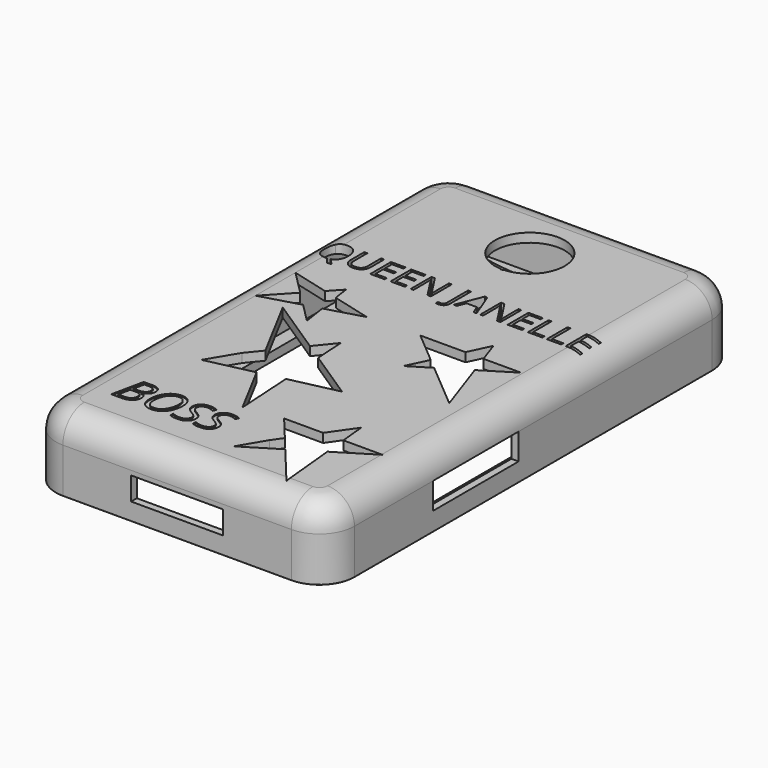
from build123d import *

# Parameters (mm, degrees)
F0_W          = 63.5
F0_H          = 112.33
F1_DEPTH      = 2
F2_W          = 63.5
F2_H          = 112.33
F3_DEPTH      = 14
F3_DEPTH_BACK = 2
F4_T1_DEPTH   = 96.7
F4_T3_DEPTH   = 145.53
F5_R          = 6.935383727
F6_T1_DEPTH   = 35.5580872669
F6_T4_ANGLE   = 90
F6_T6_ANGLE   = 90
F6_T8_ANGLE   = 90
F6_T10_ANGLE  = 90
F7_W          = 20.5546487123
F7_H          = 5.1386626437
F8_DEPTH      = 3
F9_W          = 23.8308350714
F9_H          = 5.891926311
F10_DEPTH     = 3
F11_R         = 0.0241421356
F12_W         = 98.4592325459
F12_H         = 2
F13_DEPTH     = 3
F14_SIZE2     = 2.99999
F14_SIZE      = 2.99999
F15_W         = 98.4592325459
F15_H         = 2
F16_DEPTH     = 3
F17_T1_DEPTH  = 41.9217985567
F18_W         = 49.6292325459
F18_H         = 2
F19_DEPTH     = 2
F20_T1_DEPTH  = 34.7871926215
F21_W         = 49.6292325459
F21_H         = 2
F22_DEPTH     = 2
F23_T1_DEPTH  = 68.0060422667
F24_TEXT_SIZE = 10.0512456562
F25_DEPTH     = 0.25


# Not quite as in the source:
# - a fillet or chamfer that OpenCascade refuses, or shapes differently, is made with other operations: its cross-section is extruded or revolved along the edge and cut away or added
# - a fillet or chamfer is up to 0.001 mm smaller than in the source, because OpenCascade refuses the exact size
# - Text() gives the source's letters only with a copy of the font that has no kerning and outlines rounded to 1/6400 em; it was checked with that copy


with BuildPart() as f1:
    # F0 (on Top) → F1 (new body)
    with BuildSketch(Plane.XY):
        Rectangle(F0_W, F0_H)
        Polygon((-19.5567887276, -26.5271142125), (-15.6769864261, -20.0607776642), (-13.0461571128, -16.8181271141), (-20.8500549197, -2.2136894986), (-8.0333166388, -10.6395088974), (-4.5548896305, -6.3521447591), (-4.1380456231, -13.200289134), (7.0845154114, -20.5780845135), (-3.5444898727, -22.95155196), (-2.7443135623, -36.097291857), (-9.1052395952, -24.1932729011), align=None, mode=Mode.SUBTRACT)
        Polygon((5.2739456296, -48.5126599669), (8.6364364251, -42.822279036), (10.2551206137, -40.5036243665), (5.5325948633, -34.8040238023), (14.2340888646, -34.8040238023), (18.2066168636, -29.1136484593), (18.7632836633, -34.8040238023), (27.5181401521, -34.8040238023), (19.2610861883, -39.8926750666), (20.5344967544, -52.9097691178), (12.9642616027, -43.7732775829), align=None, mode=Mode.SUBTRACT)
        Polygon((14.0059814319, -3.5149313177), (9.4123966992, -6.3521447591), (11.6904901042, -1.5602956646), (4.4979848899, 4.5113000087), (14.5769879443, 4.5113000087), (16.9133506715, 9.4257155433), (18.6099937738, 4.5113000087), (27.0008351654, 4.5113000087), (20.0847471782, 0.2395995958), (24.4142990559, -12.3011739925), align=None, mode=Mode.SUBTRACT)
        Polygon((-18.7007825335, 0.7888890234), (-27.316392865, -1.6963831149), (-21.9534791663, 4.049595339), (-27.3163933307, 9.4257155433), (-18.9805437499, 7.234883003), (-16.4529476315, 9.9430214614), (-15.9208933132, 6.4307440038), (-7.141424343, 4.1233191732), (-15.2184121265, 1.7934189192), (-14.4154893138, -3.506956622), align=None, mode=Mode.SUBTRACT)
        with BuildLine():
            add(Edge.make_bspline(
                [(-24.7315613885, 22.2938555124), (-24.029910942, 21.5008509389), (-24.029910942, 20.1051628897)],
                knots=[0, 0, 0, 1, 1, 1], degree=2))
            add(Edge.make_bspline(
                [(-24.029910942, 20.1051628897), (-24.029910942, 18.991150065), (-24.477799925, 18.2533386099)],
                knots=[0, 0, 0, 1, 1, 1], degree=2))
            add(Edge.make_bspline(
                [(-24.477799925, 18.2533386099), (-24.9256889081, 17.5155271547), (-25.7428008206, 17.2541528473)],
                knots=[0, 0, 0, 1, 1, 1], degree=2))
            Line((-25.7428008206, 17.2541528473), (-24.3636072665, 15.817862964))
            Line((-24.3636072665, 15.817862964), (-25.3431265156, 15.817862964))
            Line((-25.3431265156, 15.817862964), (-26.4723650281, 17.1272721156))
            Line((-26.4723650281, 17.1272721156), (-26.6905998867, 17.1183904644))
            add(Edge.make_bspline(
                [(-26.6905998867, 17.1183904644), (-27.9708264701, 17.1183904644), (-28.6667672837, 17.9018789829)],
                knots=[0, 0, 0, 1, 1, 1], degree=2))
            add(Edge.make_bspline(
                [(-28.6667672837, 17.9018789829), (-29.3627080973, 18.6853675015), (-29.3627080973, 20.1127757336)],
                knots=[0, 0, 0, 1, 1, 1], degree=2))
            add(Edge.make_bspline(
                [(-29.3627080973, 20.1127757336), (-29.3627080973, 21.5287646999), (-28.6648640727, 22.3078123929)],
                knots=[0, 0, 0, 1, 1, 1], degree=2))
            add(Edge.make_bspline(
                [(-28.6648640727, 22.3078123929), (-27.9670200481, 23.0868600858), (-26.6829870428, 23.0868600858)],
                knots=[0, 0, 0, 1, 1, 1], degree=2))
            add(Edge.make_bspline(
                [(-26.6829870428, 23.0868600858), (-25.4332118351, 23.0868600858), (-24.7315613885, 22.2938555124)],
                knots=[0, 0, 0, 1, 1, 1], degree=2))
        make_face(mode=Mode.SUBTRACT)
        with BuildLine():
            Line((-19.034616533, 22.9955059589), (-18.3608798475, 22.9955059589))
            Line((-18.3608798475, 22.9955059589), (-18.3608798475, 19.2449115285))
            add(Edge.make_bspline(
                [(-18.3608798475, 19.2449115285), (-18.3608798475, 18.2527042062), (-18.9597569013, 17.6855473353)],
                knots=[0, 0, 0, 1, 1, 1], degree=2))
            add(Edge.make_bspline(
                [(-18.9597569013, 17.6855473353), (-19.5586339552, 17.1183904644), (-20.6053999921, 17.1183904644)],
                knots=[0, 0, 0, 1, 1, 1], degree=2))
            add(Edge.make_bspline(
                [(-20.6053999921, 17.1183904644), (-21.652166029, 17.1183904644), (-22.2250325328, 17.6899881609)],
                knots=[0, 0, 0, 1, 1, 1], degree=2))
            add(Edge.make_bspline(
                [(-22.2250325328, 17.6899881609), (-22.7978990367, 18.2615858574), (-22.7978990367, 19.2601372163)],
                knots=[0, 0, 0, 1, 1, 1], degree=2))
            Line((-22.7978990367, 19.2601372163), (-22.7978990367, 22.9955059589))
            Line((-22.7978990367, 22.9955059589), (-22.1228935438, 22.9955059589))
            Line((-22.1228935438, 22.9955059589), (-22.1228935438, 19.2131913455))
            add(Edge.make_bspline(
                [(-22.1228935438, 19.2131913455), (-22.1228935438, 18.4874335599), (-21.7263912571, 18.0985441171)],
                knots=[0, 0, 0, 1, 1, 1], degree=2))
            add(Edge.make_bspline(
                [(-21.7263912571, 18.0985441171), (-21.3298889704, 17.7096546743), (-20.560991736, 17.7096546743)],
                knots=[0, 0, 0, 1, 1, 1], degree=2))
            add(Edge.make_bspline(
                [(-20.560991736, 17.7096546743), (-19.8276211065, 17.7096546743), (-19.4311188198, 18.1004473281)],
                knots=[0, 0, 0, 1, 1, 1], degree=2))
            add(Edge.make_bspline(
                [(-19.4311188198, 18.1004473281), (-19.034616533, 18.4912399819), (-19.034616533, 19.2208041894)],
                knots=[0, 0, 0, 1, 1, 1], degree=2))
            Line((-19.034616533, 19.2208041894), (-19.034616533, 22.9955059589))
        make_face(mode=Mode.SUBTRACT)
        Polygon((-13.595239563, 17.8010088012), (-13.595239563, 17.1983253254), (-16.8268918006, 17.1983253254), (-16.8268918006, 22.9955059589), (-13.595239563, 22.9955059589), (-13.595239563, 22.3966289051), (-16.1531551151, 22.3966289051), (-16.1531551151, 20.5289445338), (-13.7500340558, 20.5289445338), (-13.7500340558, 19.9338739019), (-16.1531551151, 19.9338739019), (-16.1531551151, 17.8010088012), align=None, mode=Mode.SUBTRACT)
        Polygon((-9.0795543201, 17.8010088012), (-9.0795543201, 17.1983253254), (-12.3112065577, 17.1983253254), (-12.3112065577, 22.9955059589), (-9.0795543201, 22.9955059589), (-9.0795543201, 22.3966289051), (-11.6374698722, 22.3966289051), (-11.6374698722, 20.5289445338), (-9.2343488128, 20.5289445338), (-9.2343488128, 19.9338739019), (-11.6374698722, 19.9338739019), (-11.6374698722, 17.8010088012), align=None, mode=Mode.SUBTRACT)
        with BuildLine():
            Line((-3.2671479987, 22.9955059589), (-3.2671479987, 17.1983253254))
            Line((-3.2671479987, 17.1983253254), (-4.0360452331, 17.1983253254))
            Line((-4.0360452331, 17.1983253254), (-7.2042571049, 22.0629325806))
            Line((-7.2042571049, 22.0629325806), (-7.2359772878, 22.0629325806))
            add(Edge.make_bspline(
                [(-7.2359772878, 22.0629325806), (-7.1725369219, 21.2064876413), (-7.1725369219, 20.4934179289)],
                knots=[0, 0, 0, 1, 1, 1], degree=2))
            Line((-7.1725369219, 20.4934179289), (-7.1725369219, 17.1983253254))
            Line((-7.1725369219, 17.1983253254), (-7.7955213148, 17.1983253254))
            Line((-7.7955213148, 17.1983253254), (-7.7955213148, 22.9955059589))
            Line((-7.7955213148, 22.9955059589), (-7.0342369243, 22.9955059589))
            Line((-7.0342369243, 22.9955059589), (-3.8736378965, 18.1499308135))
            Line((-3.8736378965, 18.1499308135), (-3.8419177136, 18.1499308135))
            add(Edge.make_bspline(
                [(-3.8419177136, 18.1499308135), (-3.8495305575, 18.2565106282), (-3.8774443185, 18.8376243796)],
                knots=[0, 0, 0, 1, 1, 1], degree=2))
            add(Edge.make_bspline(
                [(-3.8774443185, 18.8376243796), (-3.9053580794, 19.418738131), (-3.8977452355, 19.6686931725)],
                knots=[0, 0, 0, 1, 1, 1], degree=2))
            Line((-3.8977452355, 19.6686931725), (-3.8977452355, 22.9955059589))
            Line((-3.8977452355, 22.9955059589), (-3.2671479987, 22.9955059589))
        make_face(mode=Mode.SUBTRACT)
        with BuildLine():
            add(Edge.make_bspline(
                [(0.6864556025, 16.0862157116), (0.3058134073, 15.6719501224), (-0.4085251125, 15.6719501224)],
                knots=[0, 0, 0, 1, 1, 1], degree=2))
            add(Edge.make_bspline(
                [(-0.4085251125, 15.6719501224), (-0.7802856565, 15.6719501224), (-0.9947140931, 15.7785299371)],
                knots=[0, 0, 0, 1, 1, 1], degree=2))
            Line((-0.9947140931, 15.7785299371), (-0.9947140931, 16.3532996519))
            add(Edge.make_bspline(
                [(-0.9947140931, 16.3532996519), (-0.7130388687, 16.2746335983), (-0.4085251125, 16.2746335983)],
                knots=[0, 0, 0, 1, 1, 1], degree=2))
            add(Edge.make_bspline(
                [(-0.4085251125, 16.2746335983), (-0.015194844, 16.2746335983), (0.1890831341, 16.5125349703)],
                knots=[0, 0, 0, 1, 1, 1], degree=2))
            add(Edge.make_bspline(
                [(0.1890831341, 16.5125349703), (0.3933611122, 16.7504363423), (0.3933611122, 17.1983253254)],
                knots=[0, 0, 0, 1, 1, 1], degree=2))
            Line((0.3933611122, 17.1983253254), (0.3933611122, 22.9955059589))
            Line((0.3933611122, 22.9955059589), (1.0670977978, 22.9955059589))
            Line((1.0670977978, 22.9955059589), (1.0670977978, 17.2541528473))
            add(Edge.make_bspline(
                [(1.0670977978, 17.2541528473), (1.0670977978, 16.5004813008), (0.6864556025, 16.0862157116)],
                knots=[0, 0, 0, 1, 1, 1], degree=2))
        make_face(mode=Mode.SUBTRACT)
        Polygon((6.946750907, 17.1983253254), (6.2489068823, 17.1983253254), (5.5269555187, 19.0419023577), (3.2037693204, 19.0419023577), (2.490699608, 17.1983253254), (1.8080812712, 17.1983253254), (4.0995472865, 23.019613298), (4.6667041574, 23.019613298), align=None, mode=Mode.SUBTRACT)
        with BuildLine():
            Line((12.2719352184, 22.9955059589), (12.2719352184, 17.1983253254))
            Line((12.2719352184, 17.1983253254), (11.503037984, 17.1983253254))
            Line((11.503037984, 17.1983253254), (8.3348261123, 22.0629325806))
            Line((8.3348261123, 22.0629325806), (8.3031059293, 22.0629325806))
            add(Edge.make_bspline(
                [(8.3031059293, 22.0629325806), (8.3665462952, 21.2064876413), (8.3665462952, 20.4934179289)],
                knots=[0, 0, 0, 1, 1, 1], degree=2))
            Line((8.3665462952, 20.4934179289), (8.3665462952, 17.1983253254))
            Line((8.3665462952, 17.1983253254), (7.7435619023, 17.1983253254))
            Line((7.7435619023, 17.1983253254), (7.7435619023, 22.9955059589))
            Line((7.7435619023, 22.9955059589), (8.5048462928, 22.9955059589))
            Line((8.5048462928, 22.9955059589), (11.6654453207, 18.1499308135))
            Line((11.6654453207, 18.1499308135), (11.6971655036, 18.1499308135))
            add(Edge.make_bspline(
                [(11.6971655036, 18.1499308135), (11.6895526597, 18.2565106282), (11.6616388987, 18.8376243796)],
                knots=[0, 0, 0, 1, 1, 1], degree=2))
            add(Edge.make_bspline(
                [(11.6616388987, 18.8376243796), (11.6337251377, 19.418738131), (11.6413379816, 19.6686931725)],
                knots=[0, 0, 0, 1, 1, 1], degree=2))
            Line((11.6413379816, 19.6686931725), (11.6413379816, 22.9955059589))
            Line((11.6413379816, 22.9955059589), (12.2719352184, 22.9955059589))
        make_face(mode=Mode.SUBTRACT)
        Polygon((17.0972094468, 17.8010088012), (17.0972094468, 17.1983253254), (13.8655572092, 17.1983253254), (13.8655572092, 22.9955059589), (17.0972094468, 22.9955059589), (17.0972094468, 22.3966289051), (14.5392938947, 22.3966289051), (14.5392938947, 20.5289445338), (16.9424149541, 20.5289445338), (16.9424149541, 19.9338739019), (14.5392938947, 19.9338739019), (14.5392938947, 17.8010088012), align=None, mode=Mode.SUBTRACT)
        Polygon((21.6128946897, 17.1983253254), (18.3812424521, 17.1983253254), (18.3812424521, 22.9955059589), (19.0549791377, 22.9955059589), (19.0549791377, 17.8086216451), (21.6128946897, 17.8086216451), align=None, mode=Mode.SUBTRACT)
        Polygon((25.8278725984, 17.1983253254), (22.5962203607, 17.1983253254), (22.5962203607, 22.9955059589), (23.2699570463, 22.9955059589), (23.2699570463, 17.8086216451), (25.8278725984, 17.8086216451), align=None, mode=Mode.SUBTRACT)
        Polygon((30.042850507, 17.8010088012), (30.042850507, 17.1983253254), (26.8111982694, 17.1983253254), (26.8111982694, 22.9955059589), (30.042850507, 22.9955059589), (30.042850507, 22.3966289051), (27.484934955, 22.3966289051), (27.484934955, 20.5289445338), (29.8880560143, 20.5289445338), (29.8880560143, 19.9338739019), (27.484934955, 19.9338739019), (27.484934955, 17.8010088012), align=None, mode=Mode.SUBTRACT)
        with BuildLine():
            ThreePointArc((0.3612935402, 32.9422556185), (0, 32.765), (-0.3612935402, 32.9422556185))
            ThreePointArc((-0.3612935402, 32.9422556185), (-5.3783392405, 46.3566647828), (7.7889119618, 40.7227836549))
            ThreePointArc((7.7889119618, 40.7227836549), (5.6338811279, 35.3444444145), (0.3612935402, 32.9422556185))
        make_face(mode=Mode.SUBTRACT)
    extrude(amount=F1_DEPTH)

    # F2 (on face) → F3 (join, two sides)
    with BuildSketch(Plane(origin=(0, 0, 0), x_dir=(1, 0, 0), z_dir=(0, 0, -1))) as f3_sk:
        Polygon((-33.35, -57.765), (-31.75, -57.765), (31.75, -57.765), (33.35, -57.765), (33.35, -56.165), (33.35, 56.165), (33.35, 57.765), (-33.35, 57.765), (-33.35, 56.165), (-33.35, -56.165), align=None)
        Rectangle(F2_W, F2_H, mode=Mode.SUBTRACT)
    extrude(amount=F3_DEPTH)
    extrude(f3_sk.sketch, amount=-F3_DEPTH_BACK)

    # F4: fillet of radius 6 on 4 edges, made by hand

    # F4_s2 → F4_t1 (cut)
    with BuildSketch(Plane.YZ.offset(-48.35)):
        with BuildLine():
            ThreePointArc((-51.765, 2), (-56.0076406871, 0.2426406871), (-57.765, -4))
            Line((-57.765, -4), (-57.765, 2))
            Line((-57.765, 2), (-51.765, 2))
        make_face()
        with BuildLine():
            ThreePointArc((51.765, 2), (56.0076406871, 0.2426406871), (57.765, -4))
            Line((57.765, -4), (57.765, 2))
            Line((57.765, 2), (51.765, 2))
        make_face()
    extrude(amount=F4_T1_DEPTH, mode=Mode.SUBTRACT)

    # F4_s4 → F4_t3 (cut)
    with BuildSketch(Plane.XZ.offset(-72.765)):
        with BuildLine():
            ThreePointArc((27.35, 2), (31.5926406871, 0.2426406871), (33.35, -4))
            Line((33.35, -4), (33.35, 2))
            Line((33.35, 2), (27.35, 2))
        make_face()
        with BuildLine():
            ThreePointArc((-27.35, 2), (-31.5926406871, 0.2426406871), (-33.35, -4))
            Line((-33.35, -4), (-33.35, 2))
            Line((-33.35, 2), (-27.35, 2))
        make_face()
    extrude(amount=F4_T3_DEPTH, mode=Mode.SUBTRACT)

    # F5
    f5_edges = [f1.edges().sort_by_distance(p)[0] for p in [
        (31.75, -56.165, -7),
        (-31.75, -56.165, -7),
        (31.75, 56.165, -7),
        (-31.75, 56.165, -7),
    ]]
    fillet(f5_edges, radius=F5_R)

    # F6: fillet of radius 7.8232349067 on 4 edges, made by hand

    # F6_s2 → F6_t1 (cut)
    with BuildSketch(Plane.XY.offset(-33.5580872668)):
        with BuildLine():
            ThreePointArc((-25.5267650933, 57.765), (-31.0586275466, 55.4736275466), (-33.35, 49.9417650933))
            Line((-33.35, 49.9417650933), (-33.35, 57.765))
            Line((-33.35, 57.765), (-25.5267650933, 57.765))
        make_face()
        with BuildLine():
            ThreePointArc((25.5267650933, 57.765), (31.0586275466, 55.4736275466), (33.35, 49.9417650933))
            Line((33.35, 49.9417650933), (33.35, 57.765))
            Line((33.35, 57.765), (25.5267650933, 57.765))
        make_face()
        with BuildLine():
            ThreePointArc((-25.5267650933, -57.765), (-31.0586275466, -55.4736275466), (-33.35, -49.9417650933))
            Line((-33.35, -49.9417650933), (-33.35, -57.765))
            Line((-33.35, -57.765), (-25.5267650933, -57.765))
        make_face()
        with BuildLine():
            ThreePointArc((33.35, -49.9417650933), (31.0586275466, -55.4736275466), (25.5267650933, -57.765))
            Line((25.5267650933, -57.765), (33.35, -57.765))
            Line((33.35, -57.765), (33.35, -49.9417650933))
        make_face()
    extrude(amount=F6_T1_DEPTH, mode=Mode.SUBTRACT)

    # F6_s3 → F6_t4 (revolve, cut)
    with BuildSketch(Plane.YZ.offset(25.5267650933)):
        with BuildLine():
            ThreePointArc((-51.7649999999, 2), (-56.0076406871, 0.2426406871), (-57.765, -4.0000000001))
            Line((-57.765, -4.0000000001), (-57.765, 2))
            Line((-57.765, 2), (-51.7649999999, 2))
        make_face()
    revolve(axis=Axis((25.5267650933, -49.9417650933, 2), (0, 0, 1)), revolution_arc=F6_T4_ANGLE, mode=Mode.SUBTRACT)

    # F6_s5 → F6_t6 (revolve, cut)
    with BuildSketch(Plane.XZ.offset(49.9417650933)):
        with BuildLine():
            ThreePointArc((-27.3499999999, 2), (-31.5926406871, 0.2426406871), (-33.35, -4.0000000001))
            Line((-33.35, -4.0000000001), (-33.35, 2))
            Line((-33.35, 2), (-27.3499999999, 2))
        make_face()
    revolve(axis=Axis((-25.5267650933, -49.9417650933, 2), (0, 0, 1)), revolution_arc=F6_T6_ANGLE, mode=Mode.SUBTRACT)

    # F6_s7 → F6_t8 (revolve, cut)
    with BuildSketch(Plane.XZ.offset(-49.9417650933)):
        with BuildLine():
            ThreePointArc((27.3499999999, 2), (31.5926406871, 0.2426406871), (33.35, -4.0000000001))
            Line((33.35, -4.0000000001), (33.35, 2))
            Line((33.35, 2), (27.3499999999, 2))
        make_face()
    revolve(axis=Axis((25.5267650933, 49.9417650933, 2), (0, 0, 1)), revolution_arc=F6_T8_ANGLE, mode=Mode.SUBTRACT)

    # F6_s9 → F6_t10 (revolve, cut)
    with BuildSketch(Plane.YZ.offset(-25.5267650933)):
        with BuildLine():
            ThreePointArc((51.7649999999, 2), (56.0076406871, 0.2426406871), (57.765, -4.0000000001))
            Line((57.765, -4.0000000001), (57.765, 2))
            Line((57.765, 2), (51.7649999999, 2))
        make_face()
    revolve(axis=Axis((-25.5267650933, 49.9417650933, 2), (0, 0, 1)), revolution_arc=F6_T10_ANGLE, mode=Mode.SUBTRACT)

    # F7 (on face) → F8 (cut)
    with BuildSketch(Plane.XZ.offset(57.765)):
        with Locations((0, -7.5795273297)):
            Rectangle(F7_W, F7_H)
    extrude(amount=-F8_DEPTH, mode=Mode.SUBTRACT)

    # F9 (on face) → F10 (cut)
    with BuildSketch(Plane.YZ.offset(33.35)):
        with Locations((-16.0263475576, -6.9459631555)):
            Rectangle(F9_W, F9_H)
    extrude(amount=-F10_DEPTH, mode=Mode.SUBTRACT)

    # F11
    f11_edges = [f1.edges().sort_by_distance(p)[0] for p in [
        (0, 57.765, -14),
        (-31.058628, 55.473628, -14),
        (-33.35, 0, -14),
        (-31.058628, -55.473628, -14),
        (0, -57.765, -14),
        (31.058628, -55.473628, -14),
        (33.35, 0, -14),
        (31.058628, 55.473628, -14),
    ]]
    fillet(f11_edges, radius=F11_R)

    # F12 (on face) → F13 (join)
    with BuildSketch(Plane(origin=(31.75, 0, 0), x_dir=(0, -1, 0), z_dir=(-1, 0, 0))):
        with Locations((0, -13)):
            Rectangle(F12_W, F12_H)
    extrude(amount=F13_DEPTH)

    # F14 (size 3 and 3 in the source; OpenCascade refuses exactly that, so slightly less here)
    f14_edges = [f1.edges().sort_by_distance(p)[0] for p in [
        (28.75, -49.229616, -13),
        (28.75, 49.229616, -13),
    ]]
    chamfer(f14_edges, length=F14_SIZE, length2=F14_SIZE2)

    # F15 (on face) → F16 (join)
    with BuildSketch(Plane.YZ.offset(-31.75)):
        with Locations((0, -13)):
            Rectangle(F15_W, F15_H)
    extrude(amount=F16_DEPTH)

    # F17: fillet of radius 44 on 2 edges, made by hand

    # F17_s2 → F17_t1 (cut)
    with BuildSketch(Plane.XY.offset(-53.9217985567)):
        with BuildLine():
            ThreePointArc((-31.75, 49.229616273), (-29.5065033791, 41.3849352549), (-28.75, 33.2608968503))
            Line((-28.75, 33.2608968503), (-28.75, 49.229616273))
            Line((-28.75, 49.229616273), (-31.75, 49.229616273))
        make_face()
        with BuildLine():
            ThreePointArc((-31.75, -49.229616273), (-29.5065033791, -41.3849352549), (-28.75, -33.2608968503))
            Line((-28.75, -33.2608968503), (-28.75, -49.229616273))
            Line((-28.75, -49.229616273), (-31.75, -49.229616273))
        make_face()
    extrude(amount=F17_T1_DEPTH, mode=Mode.SUBTRACT)

    # F18 (on face) → F19 (join)
    with BuildSketch(Plane.XZ.offset(-56.165)):
        with Locations((0, -13)):
            Rectangle(F18_W, F18_H)
    extrude(amount=F19_DEPTH)

    # F20: fillet of radius 44 on 2 edges, made by hand

    # F20_s2 → F20_t1 (cut)
    with BuildSketch(Plane.XY.offset(-46.7871926215)):
        with BuildLine():
            ThreePointArc((-24.814616273, 56.165), (-18.3329888051, 54.6678736581), (-11.6997392244, 54.165))
            Line((-11.6997392244, 54.165), (-24.814616273, 54.165))
            Line((-24.814616273, 54.165), (-24.814616273, 56.165))
        make_face()
        with BuildLine():
            ThreePointArc((24.814616273, 56.165), (18.3329888051, 54.6678736581), (11.6997392244, 54.165))
            Line((11.6997392244, 54.165), (24.814616273, 54.165))
            Line((24.814616273, 54.165), (24.814616273, 56.165))
        make_face()
    extrude(amount=F20_T1_DEPTH, mode=Mode.SUBTRACT)

    # F21 (on face) → F22 (join)
    with BuildSketch(Plane(origin=(0, -56.165, 0), x_dir=(-1, 0, 0), z_dir=(0, 1, 0))):
        with Locations((0, -13)):
            Rectangle(F21_W, F21_H)
    extrude(amount=F22_DEPTH)

    # F23: fillet of radius 175.2719046283 on 2 edges, made by hand

    # F23_s2 → F23_t1 (cut)
    with BuildSketch(Plane.XY.offset(-80.0060422667)):
        with BuildLine():
            ThreePointArc((-24.814616273, -56.165), (-11.6512289617, -54.6657152194), (1.5878006337, -54.165))
            Line((1.5878006337, -54.165), (-24.814616273, -54.165))
            Line((-24.814616273, -54.165), (-24.814616273, -56.165))
        make_face()
        with BuildLine():
            ThreePointArc((24.814616273, -56.165), (11.6512289617, -54.6657152194), (-1.5878006337, -54.165))
            Line((-1.5878006337, -54.165), (24.814616273, -54.165))
            Line((24.814616273, -54.165), (24.814616273, -56.165))
        make_face()
    extrude(amount=F23_T1_DEPTH, mode=Mode.SUBTRACT)

    # F24 (on face) → F25 (cut)
    with BuildSketch(Plane.XY.offset(2)):
        with Locations((-24.1449766747, -46.4971400797)):
            Text('BOSS', F24_TEXT_SIZE, font='Open Sans', font_style=FontStyle.ITALIC, text_align=(TextAlign.LEFT, TextAlign.BOTTOM))
    extrude(amount=-F25_DEPTH, mode=Mode.SUBTRACT)


solid = f1.part
